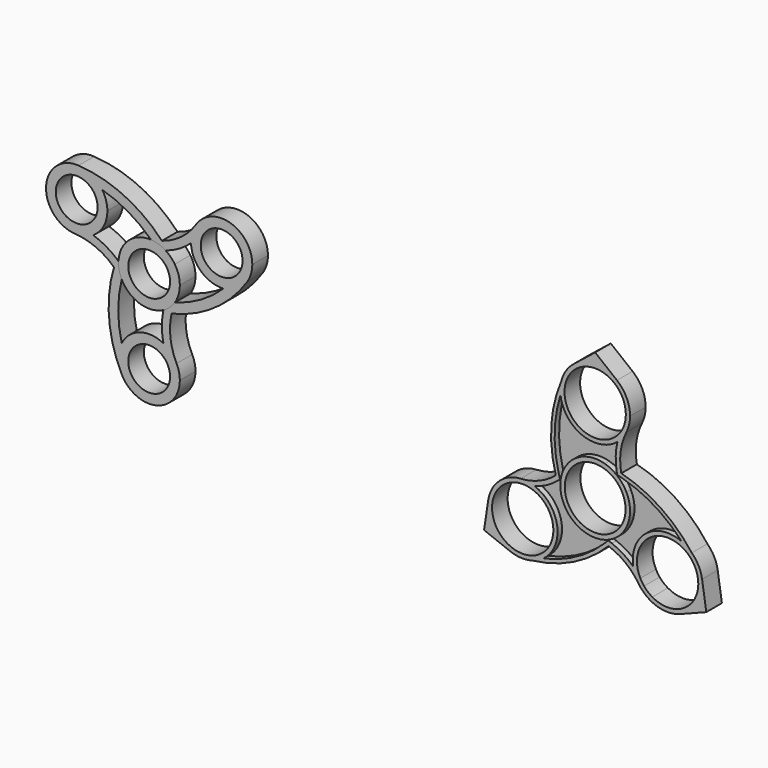
from build123d import *

# Parameters (mm, degrees)
F0_R     = 7.5
F1_DEPTH = 7
F2_DEPTH = 7
F0_R_2   = 10.9
F3_DEPTH = 5


with BuildPart() as f1:
    # F0 (on Front) → F1 (new body)
    with BuildSketch(Plane.XZ):
        with BuildLine():
            ThreePointArc((-53.6173571881, -1.7518525896), (-50.8980624665, -2.263725706), (-48.3925420942, -3.438010822))
            ThreePointArc((-48.3925420942, -3.438010822), (-48.0208333167, -3.3135242937), (-47.6510866311, -3.1833256014))
            ThreePointArc((-47.6510866311, -3.1833256014), (-48.6612372923, -1.9798547606), (-49.7132063547, -0.8127611419))
            ThreePointArc((-49.7132063547, -0.8127611419), (-51.7006557198, -1.3210314142), (-53.7260833426, -1.6465104352))
            ThreePointArc((-53.7260833426, -1.6465104352), (-53.6716717563, -1.6991314451), (-53.6173571881, -1.7518525896))
        make_face()
        with BuildLine():
            ThreePointArc((-49.7132063547, -0.8127611419), (-48.6612372923, -1.9798547606), (-47.6510866311, -3.1833256014))
            ThreePointArc((-47.6510866311, -3.1833256014), (-43.2270069865, -1.0862666914), (-39.2865137281, 1.8193571064))
            ThreePointArc((-39.2865137281, 1.8193571064), (-38.8930820127, 5.2165884842), (-37.4752941756, 8.3287978599))
            ThreePointArc((-37.4752941756, 8.3287978599), (-42.7962829401, 2.6897701484), (-49.7132063547, -0.8127611419))
        make_face()
        with BuildLine():
            ThreePointArc((-44.9512017674, -18.7514907783), (-45.0239786919, -18.7723020893), (-45.0967938264, -18.7929793129))
            ThreePointArc((-45.0967938264, -18.7929793129), (-46.8997363096, -20.8920210639), (-49.1694572375, -22.4747227981))
            ThreePointArc((-49.1694572375, -22.4747227981), (-49.2475031303, -22.8588753064), (-49.319621098, -23.2441846752))
            ThreePointArc((-49.319621098, -23.2441846752), (-47.7723094465, -22.9711039613), (-46.235592193, -22.6436188386))
            ThreePointArc((-46.235592193, -22.6436188386), (-45.6820424782, -20.6683020636), (-44.9512017674, -18.7514907783))
        make_face()
        with BuildLine():
            ThreePointArc((-27.6365950746, -8.7123288634), (-35.6733761028, -14.8021286274), (-44.9512017674, -18.7514907783))
            ThreePointArc((-44.9512017674, -18.7514907783), (-45.6820424782, -20.6683020636), (-46.235592193, -22.6436188386))
            ThreePointArc((-46.235592193, -22.6436188386), (-30.8640120209, -15.8248534989), (-19.1160317129, -3.7929793129))
            ThreePointArc((-19.1160317129, -3.7929793129), (-22.7956629442, -7.2583701681), (-27.6365950746, -8.7123288634))
        make_face()
        with BuildLine():
            ThreePointArc((-37.4752941756, 8.3287978599), (-38.8930820127, 5.2165884842), (-39.2865137281, 1.8193571064))
            ThreePointArc((-39.2865137281, 1.8193571064), (-35.6723516924, -5.8920210639), (-27.6365950746, -8.7123288634))
            ThreePointArc((-27.6365950746, -8.7123288634), (-22.7956629442, -7.2583701681), (-19.1160317129, -3.7929793129))
            ThreePointArc((-19.1160317129, -3.7929793129), (-17.7605800413, -0.8962696449), (-17.2956629442, 2.2679092735))
            ThreePointArc((-17.2956629442, 2.2679092735), (-25.1314840258, 12.8029921765), (-37.4752941756, 8.3287978599))
        make_face()
        with Locations((-28.2956629442, 2.2679092735)):
            Circle(F0_R, mode=Mode.SUBTRACT)
        with BuildLine():
            ThreePointArc((-53.7260833426, -1.6465104352), (-51.7006557198, -1.3210314142), (-49.7132063547, -0.8127611419))
            ThreePointArc((-49.7132063547, -0.8127611419), (-63.3042204474, 9.0900351135), (-79.5981193016, 13.2481474104))
            ThreePointArc((-79.5981193016, 13.2481474104), (-74.7571871713, 11.7941887151), (-71.07755594, 8.3287978599))
            ThreePointArc((-71.07755594, 8.3287978599), (-61.7852441263, 4.4136412068), (-53.7260833426, -1.6465104352))
        make_face()
        with BuildLine():
            ThreePointArc((-44.4377259568, -37.812741176), (-46.6607728253, -30.3851158769), (-46.235592193, -22.6436188386))
            ThreePointArc((-46.235592193, -22.6436188386), (-47.7723094465, -22.9711039613), (-49.319621098, -23.2441846752))
            ThreePointArc((-49.319621098, -23.2441846752), (-49.715554631, -28.1240794908), (-49.1694572375, -32.9894586549))
            ThreePointArc((-49.1694572375, -32.9894586549), (-46.4240844195, -35.028796204), (-44.4377259568, -37.812741176))
        make_face()
        with BuildLine():
            ThreePointArc((-71.07755594, 8.3287978599), (-74.7571871713, 11.7941887151), (-79.5981193016, 13.2481474104))
            ThreePointArc((-79.5981193016, 13.2481474104), (-91.2374253082, 2.9269771432), (-80.916255041, -8.7123288634))
            ThreePointArc((-80.916255041, -8.7123288634), (-77.5121087411, -8.3840644597), (-74.3733042077, -7.026170631))
            ThreePointArc((-74.3733042077, -7.026170631), (-70.6207274324, -3.0366777698), (-69.2571871713, 2.2679092735))
            ThreePointArc((-69.2571871713, 2.2679092735), (-69.7221042683, 5.4320881919), (-71.07755594, 8.3287978599))
        make_face()
        with Locations((-80.2571871713, 2.2679092735)):
            Circle(F0_R, mode=Mode.SUBTRACT)
        with BuildLine():
            ThreePointArc((-43.2764250578, -42.7320907265), (-43.5706861736, -40.2048086005), (-44.4377259568, -37.812741176))
            ThreePointArc((-44.4377259568, -37.812741176), (-46.4240844195, -35.028796204), (-49.1694572375, -32.9894586549))
            ThreePointArc((-49.1694572375, -32.9894586549), (-57.654787649, -32.263725706), (-64.1151241588, -37.812741176))
            ThreePointArc((-64.1151241588, -37.812741176), (-65.2764250578, -42.7320907265), (-64.1151241588, -47.651440277))
            ThreePointArc((-64.1151241588, -47.651440277), (-51.7491429317, -53.4378296106), (-43.2764250578, -42.7320907265))
        make_face()
        with Locations((-54.2764250578, -42.7320907265)):
            Circle(F0_R, mode=Mode.SUBTRACT)
        with BuildLine():
            ThreePointArc((-74.3733042077, -7.026170631), (-77.5121087411, -8.3840644597), (-80.916255041, -8.7123288634))
            ThreePointArc((-80.916255041, -8.7123288634), (-73.3722194079, -10.500926451), (-66.8804766256, -14.7398921989))
            ThreePointArc((-66.8804766256, -14.7398921989), (-66.3957284344, -13.2453134575), (-65.8585674442, -11.7687619029))
            ThreePointArc((-65.8585674442, -11.7687619029), (-69.8867135558, -8.9859259973), (-74.3733042077, -7.026170631))
        make_face()
        with BuildLine():
            ThreePointArc((-64.1151241588, -17.651440277), (-65.0314763972, -15.0405254095), (-65.2672758416, -12.2835385593))
            ThreePointArc((-65.2672758416, -12.2835385593), (-65.5609387263, -12.0238725794), (-65.8585674442, -11.7687619029))
            ThreePointArc((-65.8585674442, -11.7687619029), (-66.3957284344, -13.2453134575), (-66.8804766256, -14.7398921989))
            ThreePointArc((-66.8804766256, -14.7398921989), (-65.4465769753, -16.2069387016), (-64.1519900633, -17.798270966))
            ThreePointArc((-64.1519900633, -17.798270966), (-64.1336247251, -17.7248386451), (-64.1151241588, -17.651440277))
        make_face()
        with BuildLine():
            ThreePointArc((-64.1519900633, -17.798270966), (-65.4465769753, -16.2069387016), (-66.8804766256, -14.7398921989))
            ThreePointArc((-66.8804766256, -14.7398921989), (-68.6610427049, -31.4614537941), (-64.1151241588, -47.651440277))
            ThreePointArc((-64.1151241588, -47.651440277), (-65.2764250578, -42.7320907265), (-64.1151241588, -37.812741176))
            ThreePointArc((-64.1151241588, -37.812741176), (-65.3706549442, -27.8077847589), (-64.1519900633, -17.798270966))
        make_face()
        with BuildLine():
            ThreePointArc((-44.4377259568, -17.651440277), (-43.5706861736, -15.2593728525), (-43.2764250578, -12.7320907265))
            ThreePointArc((-43.2764250578, -12.7320907265), (-43.7413421548, -9.5679118081), (-45.0967938264, -6.6712021401))
            ThreePointArc((-45.0967938264, -6.6712021401), (-46.5731305353, -4.8797500882), (-48.3925420942, -3.438010822))
            ThreePointArc((-48.3925420942, -3.438010822), (-50.8980624665, -2.263725706), (-53.6173571881, -1.7518525896))
            ThreePointArc((-53.6173571881, -1.7518525896), (-54.2764250578, -1.7320907265), (-54.9354929274, -1.7518525896))
            ThreePointArc((-54.9354929274, -1.7518525896), (-60.3373136442, -3.5524594952), (-64.1151241588, -7.812741176))
            ThreePointArc((-64.1151241588, -7.812741176), (-64.9283987909, -9.9870122963), (-65.2672758416, -12.2835385593))
            ThreePointArc((-65.2672758416, -12.2835385593), (-65.0314763972, -15.0405254095), (-64.1151241588, -17.651440277))
            ThreePointArc((-64.1151241588, -17.651440277), (-63.8027044994, -18.2320907265), (-63.4560562891, -18.7929793129))
            ThreePointArc((-63.4560562891, -18.7929793129), (-59.1957746083, -22.5707898275), (-53.6173571881, -23.7123288634))
            ThreePointArc((-53.6173571881, -23.7123288634), (-51.3277458471, -23.3295097949), (-49.1694572375, -22.4747227981))
            ThreePointArc((-49.1694572375, -22.4747227981), (-46.8997363096, -20.8920210639), (-45.0967938264, -18.7929793129))
            ThreePointArc((-45.0967938264, -18.7929793129), (-44.7501456161, -18.2320907265), (-44.4377259568, -17.651440277))
        make_face()
        with Locations((-54.2764250578, -12.7320907265)):
            Circle(F0_R, mode=Mode.SUBTRACT)
    extrude(amount=F1_DEPTH)


with BuildPart() as f1b:
    # F0 (on Front) → F1, piece 2 (new body)
    with BuildSketch(Plane.XZ):
        with BuildLine():
            ThreePointArc((113.2901036685, -20.2251223841), (113.4145637461, -20.9117406905), (113.5601241099, -21.5941974218))
            ThreePointArc((113.5601241099, -21.5941974218), (114.4419800019, -21.8056031634), (115.3193491866, -22.034918482))
            ThreePointArc((115.3193491866, -22.034918482), (115.1420860534, -21.3333227671), (114.989053465, -20.6260464472))
            ThreePointArc((114.989053465, -20.6260464472), (114.141488051, -20.4174928136), (113.2901036685, -20.2251223841))
        make_face()
        with BuildLine():
            ThreePointArc((113.6417849809, -11.123598484), (113.0035342504, -15.6564929886), (113.2901036685, -20.2251223841))
            ThreePointArc((113.2901036685, -20.2251223841), (114.141488051, -20.4174928136), (114.989053465, -20.6260464472))
            ThreePointArc((114.989053465, -20.6260464472), (114.7749384437, -13.7221170116), (116.8080124932, -7.1208522234))
            ThreePointArc((116.8080124932, -7.1208522234), (117.7932836947, -4.4025953564), (118.1276708841, -1.5306857228))
            ThreePointArc((118.1276708841, -1.5306857228), (116.8949207212, 3.8821768385), (113.4398179068, 8.2274062472))
            ThreePointArc((113.4398179068, 8.2274062472), (105.6276708841, 10.9693142772), (97.8155238614, 8.2274062472))
            ThreePointArc((97.8155238614, 8.2274062472), (95.0980135598, 5.2055087987), (93.4935622624, 1.4715481048))
            ThreePointArc((93.4935622624, 1.4715481048), (89.9070791367, -13.5321823635), (91.503284962, -28.8758102311))
            ThreePointArc((91.503284962, -28.8758102311), (92.0392879282, -28.389641962), (92.558256074, -27.885329728))
            ThreePointArc((92.558256074, -27.885329728), (91.1017738419, -15.3701146731), (93.2082555904, -2.9477685578))
            ThreePointArc((93.2082555904, -2.9477685578), (100.9841034619, -13.1361707017), (113.6417849809, -11.123598484))
        make_face()
        with BuildLine():
            ThreePointArc((114.8625762594, -7.5070159271), (95.0781694948, 1.585083915), (116.6276708841, -1.5306857228))
            ThreePointArc((116.6276708841, -1.5306857228), (116.4568463207, -3.4617370849), (115.9496782727, -5.3328119005))
            ThreePointArc((115.9496782727, -5.3328119005), (115.4663699851, -6.4500352733), (114.8625762594, -7.5070159271))
        make_face(mode=Mode.SUBTRACT)
        with BuildLine():
            ThreePointArc((114.989053465, -20.6260464472), (115.1420860534, -21.3333227671), (115.3193491866, -22.034918482))
            ThreePointArc((115.3193491866, -22.034918482), (126.886084474, -27.0311753964), (136.5909109102, -35.0666151608))
            ThreePointArc((136.5909109102, -35.0666151608), (123.8795718938, -36.7064958816), (119.2936698018, -48.6746557389))
            ThreePointArc((119.2936698018, -48.6746557389), (115.6871933734, -45.85546714), (111.5873595473, -43.8193288382))
            ThreePointArc((111.5873595473, -43.8193288382), (110.9950696772, -44.4604641271), (110.3906742255, -45.0902004902))
            ThreePointArc((110.3906742255, -45.0902004902), (116.4767100133, -48.3567361602), (121.1770359922, -53.418062329))
            ThreePointArc((121.1770359922, -53.418062329), (123.0384798923, -55.6304606526), (125.3584329977, -57.3560032701))
            ThreePointArc((125.3584329977, -57.3560032701), (130.6624845644, -58.9948415932), (136.1531150248, -58.1752494876))
            ThreePointArc((136.1531150248, -58.1752494876), (142.433750545, -52.7806857228), (143.9652620475, -44.6442139281))
            ThreePointArc((143.9652620475, -44.6442139281), (142.7069772403, -40.7798322475), (140.2754980714, -37.5233563179))
            ThreePointArc((140.2754980714, -37.5233563179), (129.0751278972, -26.9155055867), (114.989053465, -20.6260464472))
        make_face()
        with BuildLine():
            ThreePointArc((142.6084329977, -46.5306857228), (137.1084329977, -56.0569651645), (126.1084329977, -56.0569651645))
            ThreePointArc((126.1084329977, -56.0569651645), (124.5215057438, -54.9435010719), (123.1546914451, -53.5687432505))
            ThreePointArc((123.1546914451, -53.5687432505), (122.4288017663, -52.5915743092), (121.8153265318, -51.5401832772))
            ThreePointArc((121.8153265318, -51.5401832772), (129.0320179617, -35.8366647035), (142.6084329977, -46.5306857228))
        make_face(mode=Mode.SUBTRACT)
        with BuildLine():
            ThreePointArc((110.3906742255, -45.0902004902), (110.9950696772, -44.4604641271), (111.5873595473, -43.8193288382))
            ThreePointArc((111.5873595473, -43.8193288382), (110.9305006125, -43.583805274), (110.2666955643, -43.3686358812))
            ThreePointArc((110.2666955643, -43.3686358812), (109.6426848757, -44.0266426153), (109.0054073918, -44.6718089585))
            ThreePointArc((109.0054073918, -44.6718089585), (109.7016386708, -44.8690924394), (110.3906742255, -45.0902004902))
        make_face()
        with BuildLine():
            ThreePointArc((93.0561929781, -29.6292238655), (92.7983477749, -28.7598113898), (92.558256074, -27.885329728))
            ThreePointArc((92.558256074, -27.885329728), (92.0392879282, -28.389641962), (91.503284962, -28.8758102311))
            ThreePointArc((91.503284962, -28.8758102311), (91.7464549242, -29.7141002277), (92.0055494366, -30.5476059461))
            ThreePointArc((92.0055494366, -30.5476059461), (92.5379482938, -30.096511204), (93.0561929781, -29.6292238655))
        make_face()
        with BuildLine():
            ThreePointArc((83.1139523186, -58.5402489554), (97.9008056186, -54.1443692183), (110.3906742255, -45.0902004902))
            ThreePointArc((110.3906742255, -45.0902004902), (109.7016386708, -44.8690924394), (109.0054073918, -44.6718089585))
            ThreePointArc((109.0054073918, -44.6718089585), (98.8951543365, -52.190767099), (87.0838461519, -56.5776734499))
            ThreePointArc((87.0838461519, -56.5776734499), (92.0193372967, -44.7493905852), (83.9475578697, -34.7938029456))
            ThreePointArc((83.9475578697, -34.7938029456), (88.1922850286, -33.0800970399), (92.0055494366, -30.5476059461))
            ThreePointArc((92.0055494366, -30.5476059461), (91.7464549242, -29.7141002277), (91.503284962, -28.8758102311))
            ThreePointArc((91.503284962, -28.8758102311), (85.6313641954, -32.5132039966), (78.897964167, -34.0531426161))
            ThreePointArc((78.897964167, -34.0531426161), (76.0512490654, -34.5590011595), (73.3969087706, -35.7053681755))
            ThreePointArc((73.3969087706, -35.7053681755), (69.3256073667, -39.4793924138), (67.2900797207, -44.6442139281))
            ThreePointArc((67.2900797207, -44.6442139281), (68.8215912233, -52.7806857228), (75.1022267434, -58.1752494876))
            ThreePointArc((75.1022267434, -58.1752494876), (79.0780218523, -59.0177337196), (83.1139523186, -58.5402489554))
        make_face()
        with BuildLine():
            ThreePointArc((90.6469087706, -46.5306857228), (74.1469087706, -56.0569651645), (74.1469087706, -37.0044062812))
            ThreePointArc((74.1469087706, -37.0044062812), (75.9046605879, -36.1868190116), (77.7786429346, -35.6905020175))
            ThreePointArc((77.7786429346, -35.6905020175), (78.9878409009, -35.5504475859), (80.2051098612, -35.5448579642))
            ThreePointArc((80.2051098612, -35.5448579642), (87.619995124, -38.9524343413), (90.6469087706, -46.5306857228))
        make_face(mode=Mode.SUBTRACT)
        with BuildLine():
            Line((145.4755362958, -54.5368615449), (143.9652620475, -44.6442139281))
            ThreePointArc((143.9652620475, -44.6442139281), (142.433750545, -52.7806857228), (136.1531150248, -58.1752494876))
            Line((136.1531150248, -58.1752494876), (145.4755362958, -54.5368615449))
        make_face()
        with BuildLine():
            ThreePointArc((97.8155238614, 8.2274062472), (105.6276708841, 10.9693142772), (113.4398179068, 8.2274062472))
            Line((113.4398179068, 8.2274062472), (105.6276708841, 14.4816659213))
            Line((105.6276708841, 14.4816659213), (97.8155238614, 8.2274062472))
        make_face()
        with BuildLine():
            Line((65.7798054725, -54.5368615449), (75.1022267434, -58.1752494876))
            ThreePointArc((75.1022267434, -58.1752494876), (68.8215912233, -52.7806857228), (67.2900797207, -44.6442139281))
            Line((67.2900797207, -44.6442139281), (65.7798054725, -54.5368615449))
        make_face()
    extrude(amount=F1_DEPTH)


with BuildPart() as f2:
    # F0 (on Front) → F2 (new body)
    with BuildSketch(Plane.XZ):
        with BuildLine():
            ThreePointArc((-53.6173571881, -1.7518525896), (-50.8980624665, -2.263725706), (-48.3925420942, -3.438010822))
            ThreePointArc((-48.3925420942, -3.438010822), (-48.0208333167, -3.3135242937), (-47.6510866311, -3.1833256014))
            ThreePointArc((-47.6510866311, -3.1833256014), (-48.6612372923, -1.9798547606), (-49.7132063547, -0.8127611419))
            ThreePointArc((-49.7132063547, -0.8127611419), (-51.7006557198, -1.3210314142), (-53.7260833426, -1.6465104352))
            ThreePointArc((-53.7260833426, -1.6465104352), (-53.6716717563, -1.6991314451), (-53.6173571881, -1.7518525896))
        make_face()
        with BuildLine():
            ThreePointArc((-49.7132063547, -0.8127611419), (-48.6612372923, -1.9798547606), (-47.6510866311, -3.1833256014))
            ThreePointArc((-47.6510866311, -3.1833256014), (-43.2270069865, -1.0862666914), (-39.2865137281, 1.8193571064))
            ThreePointArc((-39.2865137281, 1.8193571064), (-38.8930820127, 5.2165884842), (-37.4752941756, 8.3287978599))
            ThreePointArc((-37.4752941756, 8.3287978599), (-42.7962829401, 2.6897701484), (-49.7132063547, -0.8127611419))
        make_face()
        with BuildLine():
            ThreePointArc((-44.9512017674, -18.7514907783), (-45.0239786919, -18.7723020893), (-45.0967938264, -18.7929793129))
            ThreePointArc((-45.0967938264, -18.7929793129), (-46.8997363096, -20.8920210639), (-49.1694572375, -22.4747227981))
            ThreePointArc((-49.1694572375, -22.4747227981), (-49.2475031303, -22.8588753064), (-49.319621098, -23.2441846752))
            ThreePointArc((-49.319621098, -23.2441846752), (-47.7723094465, -22.9711039613), (-46.235592193, -22.6436188386))
            ThreePointArc((-46.235592193, -22.6436188386), (-45.6820424782, -20.6683020636), (-44.9512017674, -18.7514907783))
        make_face()
        with BuildLine():
            ThreePointArc((-27.6365950746, -8.7123288634), (-35.6733761028, -14.8021286274), (-44.9512017674, -18.7514907783))
            ThreePointArc((-44.9512017674, -18.7514907783), (-45.6820424782, -20.6683020636), (-46.235592193, -22.6436188386))
            ThreePointArc((-46.235592193, -22.6436188386), (-30.8640120209, -15.8248534989), (-19.1160317129, -3.7929793129))
            ThreePointArc((-19.1160317129, -3.7929793129), (-22.7956629442, -7.2583701681), (-27.6365950746, -8.7123288634))
        make_face()
        with BuildLine():
            ThreePointArc((-37.4752941756, 8.3287978599), (-38.8930820127, 5.2165884842), (-39.2865137281, 1.8193571064))
            ThreePointArc((-39.2865137281, 1.8193571064), (-35.6723516924, -5.8920210639), (-27.6365950746, -8.7123288634))
            ThreePointArc((-27.6365950746, -8.7123288634), (-22.7956629442, -7.2583701681), (-19.1160317129, -3.7929793129))
            ThreePointArc((-19.1160317129, -3.7929793129), (-17.7605800413, -0.8962696449), (-17.2956629442, 2.2679092735))
            ThreePointArc((-17.2956629442, 2.2679092735), (-25.1314840258, 12.8029921765), (-37.4752941756, 8.3287978599))
        make_face()
        with Locations((-28.2956629442, 2.2679092735)):
            Circle(F0_R, mode=Mode.SUBTRACT)
        with BuildLine():
            ThreePointArc((-53.7260833426, -1.6465104352), (-51.7006557198, -1.3210314142), (-49.7132063547, -0.8127611419))
            ThreePointArc((-49.7132063547, -0.8127611419), (-63.3042204474, 9.0900351135), (-79.5981193016, 13.2481474104))
            ThreePointArc((-79.5981193016, 13.2481474104), (-74.7571871713, 11.7941887151), (-71.07755594, 8.3287978599))
            ThreePointArc((-71.07755594, 8.3287978599), (-61.7852441263, 4.4136412068), (-53.7260833426, -1.6465104352))
        make_face()
        with BuildLine():
            ThreePointArc((-44.4377259568, -37.812741176), (-46.6607728253, -30.3851158769), (-46.235592193, -22.6436188386))
            ThreePointArc((-46.235592193, -22.6436188386), (-47.7723094465, -22.9711039613), (-49.319621098, -23.2441846752))
            ThreePointArc((-49.319621098, -23.2441846752), (-49.715554631, -28.1240794908), (-49.1694572375, -32.9894586549))
            ThreePointArc((-49.1694572375, -32.9894586549), (-46.4240844195, -35.028796204), (-44.4377259568, -37.812741176))
        make_face()
        with BuildLine():
            ThreePointArc((-71.07755594, 8.3287978599), (-74.7571871713, 11.7941887151), (-79.5981193016, 13.2481474104))
            ThreePointArc((-79.5981193016, 13.2481474104), (-91.2374253082, 2.9269771432), (-80.916255041, -8.7123288634))
            ThreePointArc((-80.916255041, -8.7123288634), (-77.5121087411, -8.3840644597), (-74.3733042077, -7.026170631))
            ThreePointArc((-74.3733042077, -7.026170631), (-70.6207274324, -3.0366777698), (-69.2571871713, 2.2679092735))
            ThreePointArc((-69.2571871713, 2.2679092735), (-69.7221042683, 5.4320881919), (-71.07755594, 8.3287978599))
        make_face()
        with Locations((-80.2571871713, 2.2679092735)):
            Circle(F0_R, mode=Mode.SUBTRACT)
        with BuildLine():
            ThreePointArc((-43.2764250578, -42.7320907265), (-43.5706861736, -40.2048086005), (-44.4377259568, -37.812741176))
            ThreePointArc((-44.4377259568, -37.812741176), (-46.4240844195, -35.028796204), (-49.1694572375, -32.9894586549))
            ThreePointArc((-49.1694572375, -32.9894586549), (-57.654787649, -32.263725706), (-64.1151241588, -37.812741176))
            ThreePointArc((-64.1151241588, -37.812741176), (-65.2764250578, -42.7320907265), (-64.1151241588, -47.651440277))
            ThreePointArc((-64.1151241588, -47.651440277), (-51.7491429317, -53.4378296106), (-43.2764250578, -42.7320907265))
        make_face()
        with Locations((-54.2764250578, -42.7320907265)):
            Circle(F0_R, mode=Mode.SUBTRACT)
        with BuildLine():
            ThreePointArc((-74.3733042077, -7.026170631), (-77.5121087411, -8.3840644597), (-80.916255041, -8.7123288634))
            ThreePointArc((-80.916255041, -8.7123288634), (-73.3722194079, -10.500926451), (-66.8804766256, -14.7398921989))
            ThreePointArc((-66.8804766256, -14.7398921989), (-66.3957284344, -13.2453134575), (-65.8585674442, -11.7687619029))
            ThreePointArc((-65.8585674442, -11.7687619029), (-69.8867135558, -8.9859259973), (-74.3733042077, -7.026170631))
        make_face()
        with BuildLine():
            ThreePointArc((-64.1151241588, -17.651440277), (-65.0314763972, -15.0405254095), (-65.2672758416, -12.2835385593))
            ThreePointArc((-65.2672758416, -12.2835385593), (-65.5609387263, -12.0238725794), (-65.8585674442, -11.7687619029))
            ThreePointArc((-65.8585674442, -11.7687619029), (-66.3957284344, -13.2453134575), (-66.8804766256, -14.7398921989))
            ThreePointArc((-66.8804766256, -14.7398921989), (-65.4465769753, -16.2069387016), (-64.1519900633, -17.798270966))
            ThreePointArc((-64.1519900633, -17.798270966), (-64.1336247251, -17.7248386451), (-64.1151241588, -17.651440277))
        make_face()
        with BuildLine():
            ThreePointArc((-64.1519900633, -17.798270966), (-65.4465769753, -16.2069387016), (-66.8804766256, -14.7398921989))
            ThreePointArc((-66.8804766256, -14.7398921989), (-68.6610427049, -31.4614537941), (-64.1151241588, -47.651440277))
            ThreePointArc((-64.1151241588, -47.651440277), (-65.2764250578, -42.7320907265), (-64.1151241588, -37.812741176))
            ThreePointArc((-64.1151241588, -37.812741176), (-65.3706549442, -27.8077847589), (-64.1519900633, -17.798270966))
        make_face()
    extrude(amount=F2_DEPTH)


with BuildPart() as f2b:
    # F0 (on Front) → F2, piece 2 (new body)
    with BuildSketch(Plane.XZ):
        with BuildLine():
            ThreePointArc((113.2901036685, -20.2251223841), (113.4145637461, -20.9117406905), (113.5601241099, -21.5941974218))
            ThreePointArc((113.5601241099, -21.5941974218), (114.4419800019, -21.8056031634), (115.3193491866, -22.034918482))
            ThreePointArc((115.3193491866, -22.034918482), (115.1420860534, -21.3333227671), (114.989053465, -20.6260464472))
            ThreePointArc((114.989053465, -20.6260464472), (114.141488051, -20.4174928136), (113.2901036685, -20.2251223841))
        make_face()
        with BuildLine():
            ThreePointArc((113.6417849809, -11.123598484), (113.0035342504, -15.6564929886), (113.2901036685, -20.2251223841))
            ThreePointArc((113.2901036685, -20.2251223841), (114.141488051, -20.4174928136), (114.989053465, -20.6260464472))
            ThreePointArc((114.989053465, -20.6260464472), (114.7749384437, -13.7221170116), (116.8080124932, -7.1208522234))
            ThreePointArc((116.8080124932, -7.1208522234), (117.7932836947, -4.4025953564), (118.1276708841, -1.5306857228))
            ThreePointArc((118.1276708841, -1.5306857228), (116.8949207212, 3.8821768385), (113.4398179068, 8.2274062472))
            ThreePointArc((113.4398179068, 8.2274062472), (105.6276708841, 10.9693142772), (97.8155238614, 8.2274062472))
            ThreePointArc((97.8155238614, 8.2274062472), (95.0980135598, 5.2055087987), (93.4935622624, 1.4715481048))
            ThreePointArc((93.4935622624, 1.4715481048), (89.9070791367, -13.5321823635), (91.503284962, -28.8758102311))
            ThreePointArc((91.503284962, -28.8758102311), (92.0392879282, -28.389641962), (92.558256074, -27.885329728))
            ThreePointArc((92.558256074, -27.885329728), (91.1017738419, -15.3701146731), (93.2082555904, -2.9477685578))
            ThreePointArc((93.2082555904, -2.9477685578), (100.9841034619, -13.1361707017), (113.6417849809, -11.123598484))
        make_face()
        with BuildLine():
            ThreePointArc((114.8625762594, -7.5070159271), (95.0781694948, 1.585083915), (116.6276708841, -1.5306857228))
            ThreePointArc((116.6276708841, -1.5306857228), (116.4568463207, -3.4617370849), (115.9496782727, -5.3328119005))
            ThreePointArc((115.9496782727, -5.3328119005), (115.4663699851, -6.4500352733), (114.8625762594, -7.5070159271))
        make_face(mode=Mode.SUBTRACT)
        with BuildLine():
            ThreePointArc((114.989053465, -20.6260464472), (115.1420860534, -21.3333227671), (115.3193491866, -22.034918482))
            ThreePointArc((115.3193491866, -22.034918482), (126.886084474, -27.0311753964), (136.5909109102, -35.0666151608))
            ThreePointArc((136.5909109102, -35.0666151608), (123.8795718938, -36.7064958816), (119.2936698018, -48.6746557389))
            ThreePointArc((119.2936698018, -48.6746557389), (115.6871933734, -45.85546714), (111.5873595473, -43.8193288382))
            ThreePointArc((111.5873595473, -43.8193288382), (110.9950696772, -44.4604641271), (110.3906742255, -45.0902004902))
            ThreePointArc((110.3906742255, -45.0902004902), (116.4767100133, -48.3567361602), (121.1770359922, -53.418062329))
            ThreePointArc((121.1770359922, -53.418062329), (123.0384798923, -55.6304606526), (125.3584329977, -57.3560032701))
            ThreePointArc((125.3584329977, -57.3560032701), (130.6624845644, -58.9948415932), (136.1531150248, -58.1752494876))
            ThreePointArc((136.1531150248, -58.1752494876), (142.433750545, -52.7806857228), (143.9652620475, -44.6442139281))
            ThreePointArc((143.9652620475, -44.6442139281), (142.7069772403, -40.7798322475), (140.2754980714, -37.5233563179))
            ThreePointArc((140.2754980714, -37.5233563179), (129.0751278972, -26.9155055867), (114.989053465, -20.6260464472))
        make_face()
        with BuildLine():
            ThreePointArc((142.6084329977, -46.5306857228), (137.1084329977, -56.0569651645), (126.1084329977, -56.0569651645))
            ThreePointArc((126.1084329977, -56.0569651645), (124.5215057438, -54.9435010719), (123.1546914451, -53.5687432505))
            ThreePointArc((123.1546914451, -53.5687432505), (122.4288017663, -52.5915743092), (121.8153265318, -51.5401832772))
            ThreePointArc((121.8153265318, -51.5401832772), (129.0320179617, -35.8366647035), (142.6084329977, -46.5306857228))
        make_face(mode=Mode.SUBTRACT)
        with BuildLine():
            ThreePointArc((110.3906742255, -45.0902004902), (110.9950696772, -44.4604641271), (111.5873595473, -43.8193288382))
            ThreePointArc((111.5873595473, -43.8193288382), (110.9305006125, -43.583805274), (110.2666955643, -43.3686358812))
            ThreePointArc((110.2666955643, -43.3686358812), (109.6426848757, -44.0266426153), (109.0054073918, -44.6718089585))
            ThreePointArc((109.0054073918, -44.6718089585), (109.7016386708, -44.8690924394), (110.3906742255, -45.0902004902))
        make_face()
        with BuildLine():
            ThreePointArc((93.0561929781, -29.6292238655), (92.7983477749, -28.7598113898), (92.558256074, -27.885329728))
            ThreePointArc((92.558256074, -27.885329728), (92.0392879282, -28.389641962), (91.503284962, -28.8758102311))
            ThreePointArc((91.503284962, -28.8758102311), (91.7464549242, -29.7141002277), (92.0055494366, -30.5476059461))
            ThreePointArc((92.0055494366, -30.5476059461), (92.5379482938, -30.096511204), (93.0561929781, -29.6292238655))
        make_face()
        with BuildLine():
            ThreePointArc((83.1139523186, -58.5402489554), (97.9008056186, -54.1443692183), (110.3906742255, -45.0902004902))
            ThreePointArc((110.3906742255, -45.0902004902), (109.7016386708, -44.8690924394), (109.0054073918, -44.6718089585))
            ThreePointArc((109.0054073918, -44.6718089585), (98.8951543365, -52.190767099), (87.0838461519, -56.5776734499))
            ThreePointArc((87.0838461519, -56.5776734499), (92.0193372967, -44.7493905852), (83.9475578697, -34.7938029456))
            ThreePointArc((83.9475578697, -34.7938029456), (88.1922850286, -33.0800970399), (92.0055494366, -30.5476059461))
            ThreePointArc((92.0055494366, -30.5476059461), (91.7464549242, -29.7141002277), (91.503284962, -28.8758102311))
            ThreePointArc((91.503284962, -28.8758102311), (85.6313641954, -32.5132039966), (78.897964167, -34.0531426161))
            ThreePointArc((78.897964167, -34.0531426161), (76.0512490654, -34.5590011595), (73.3969087706, -35.7053681755))
            ThreePointArc((73.3969087706, -35.7053681755), (69.3256073667, -39.4793924138), (67.2900797207, -44.6442139281))
            ThreePointArc((67.2900797207, -44.6442139281), (68.8215912233, -52.7806857228), (75.1022267434, -58.1752494876))
            ThreePointArc((75.1022267434, -58.1752494876), (79.0780218523, -59.0177337196), (83.1139523186, -58.5402489554))
        make_face()
        with BuildLine():
            ThreePointArc((90.6469087706, -46.5306857228), (74.1469087706, -56.0569651645), (74.1469087706, -37.0044062812))
            ThreePointArc((74.1469087706, -37.0044062812), (75.9046605879, -36.1868190116), (77.7786429346, -35.6905020175))
            ThreePointArc((77.7786429346, -35.6905020175), (78.9878409009, -35.5504475859), (80.2051098612, -35.5448579642))
            ThreePointArc((80.2051098612, -35.5448579642), (87.619995124, -38.9524343413), (90.6469087706, -46.5306857228))
        make_face(mode=Mode.SUBTRACT)
        with BuildLine():
            Line((145.4755362958, -54.5368615449), (143.9652620475, -44.6442139281))
            ThreePointArc((143.9652620475, -44.6442139281), (142.433750545, -52.7806857228), (136.1531150248, -58.1752494876))
            Line((136.1531150248, -58.1752494876), (145.4755362958, -54.5368615449))
        make_face()
        with BuildLine():
            ThreePointArc((97.8155238614, 8.2274062472), (105.6276708841, 10.9693142772), (113.4398179068, 8.2274062472))
            Line((113.4398179068, 8.2274062472), (105.6276708841, 14.4816659213))
            Line((105.6276708841, 14.4816659213), (97.8155238614, 8.2274062472))
        make_face()
        with BuildLine():
            Line((65.7798054725, -54.5368615449), (75.1022267434, -58.1752494876))
            ThreePointArc((75.1022267434, -58.1752494876), (68.8215912233, -52.7806857228), (67.2900797207, -44.6442139281))
            Line((67.2900797207, -44.6442139281), (65.7798054725, -54.5368615449))
        make_face()
    extrude(amount=F2_DEPTH)


with BuildPart() as f2c:
    # F0 (on Front) → F2, piece 3 (new body)
    with BuildSketch(Plane.XZ):
        with BuildLine():
            ThreePointArc((116.8080107716, -25.9405157791), (115.4313565918, -23.7758326265), (113.6417849809, -21.9377729616))
            ThreePointArc((113.6417849809, -21.9377729616), (113.356531988, -21.7064958816), (113.0646082654, -21.4836979958))
            ThreePointArc((113.0646082654, -21.4836979958), (111.16726705, -20.3252016048), (109.0947144322, -19.5211224903))
            ThreePointArc((109.0947144322, -19.5211224903), (101.3050826153, -19.8018652085), (95.1962717576, -24.6433123292))
            ThreePointArc((95.1962717576, -24.6433123292), (94.0099282463, -26.9178713975), (93.3129076883, -29.3867157068))
            ThreePointArc((93.3129076883, -29.3867157068), (93.2552423581, -29.7493905852), (93.2082555904, -30.1136028878))
            ThreePointArc((93.2082555904, -30.1136028878), (93.1536388933, -32.3359967755), (93.4935622624, -34.5329195505))
            ThreePointArc((93.4935622624, -34.5329195505), (97.6315084967, -41.1385672309), (104.8787301231, -44.0082290602))
            ThreePointArc((104.8787301231, -44.0082290602), (107.4417278144, -43.8983531445), (109.9283199832, -43.2675685001))
            ThreePointArc((109.9283199832, -43.2675685001), (110.2712383063, -43.1361707017), (110.6101487966, -42.9947562849))
            ThreePointArc((110.6101487966, -42.9947562849), (112.5621067091, -41.9308587882), (114.2947359578, -40.5380151277))
            ThreePointArc((114.2947359578, -40.5380151277), (117.9464215404, -33.6516247291), (116.8080107716, -25.9405157791))
        make_face()
        with Locations((105.6276708841, -31.5306857228)):
            Circle(F0_R_2, mode=Mode.SUBTRACT)
    extrude(amount=F2_DEPTH)


with BuildPart() as f3:
    # F0 (on Front) → F3 (new body)
    with BuildSketch(Plane.XZ):
        with BuildLine():
            ThreePointArc((113.5601241099, -21.5941974218), (113.6002846637, -21.7661444089), (113.6417849809, -21.9377729616))
            ThreePointArc((113.6417849809, -21.9377729616), (115.4313565918, -23.7758326265), (116.8080107716, -25.9405157791))
            ThreePointArc((116.8080107716, -25.9405157791), (115.9664612903, -24.0247731085), (115.3193491866, -22.034918482))
            ThreePointArc((115.3193491866, -22.034918482), (114.4419800019, -21.8056031634), (113.5601241099, -21.5941974218))
        make_face()
        with BuildLine():
            ThreePointArc((115.3193491866, -22.034918482), (115.9664612903, -24.0247731085), (116.8080107716, -25.9405157791))
            ThreePointArc((116.8080107716, -25.9405157791), (117.9464215404, -33.6516247291), (114.2947359578, -40.5380151277))
            ThreePointArc((114.2947359578, -40.5380151277), (112.9791499731, -42.2101097125), (111.5873595473, -43.8193288382))
            ThreePointArc((111.5873595473, -43.8193288382), (115.6871933734, -45.85546714), (119.2936698018, -48.6746557389))
            ThreePointArc((119.2936698018, -48.6746557389), (123.8795718938, -36.7064958816), (136.5909109102, -35.0666151608))
            ThreePointArc((136.5909109102, -35.0666151608), (126.886084474, -27.0311753964), (115.3193491866, -22.034918482))
        make_face()
        with BuildLine():
            ThreePointArc((111.5873595473, -43.8193288382), (112.9791499731, -42.2101097125), (114.2947359578, -40.5380151277))
            ThreePointArc((114.2947359578, -40.5380151277), (112.5621067091, -41.9308587882), (110.6101487966, -42.9947562849))
            ThreePointArc((110.6101487966, -42.9947562849), (110.4389548786, -43.1821854301), (110.2666955643, -43.3686358812))
            ThreePointArc((110.2666955643, -43.3686358812), (110.9305006125, -43.583805274), (111.5873595473, -43.8193288382))
        make_face()
    extrude(amount=F3_DEPTH)


with BuildPart() as f3b:
    # F0 (on Front) → F3, piece 2 (new body)
    with BuildSketch(Plane.XZ):
        with BuildLine():
            ThreePointArc((109.0947144322, -19.5211224903), (111.16726705, -20.3252016048), (113.0646082654, -21.4836979958))
            ThreePointArc((113.0646082654, -21.4836979958), (113.3125236256, -21.5382417051), (113.5601241099, -21.5941974218))
            ThreePointArc((113.5601241099, -21.5941974218), (113.4145637461, -20.9117406905), (113.2901036685, -20.2251223841))
            ThreePointArc((113.2901036685, -20.2251223841), (111.2005838125, -19.8244060816), (109.0947144322, -19.5211224903))
        make_face()
        with BuildLine():
            ThreePointArc((95.1962717576, -24.6433123292), (101.3050826153, -19.8018652085), (109.0947144322, -19.5211224903))
            ThreePointArc((109.0947144322, -19.5211224903), (111.2005838125, -19.8244060816), (113.2901036685, -20.2251223841))
            ThreePointArc((113.2901036685, -20.2251223841), (113.0035342504, -15.6564929886), (113.6417849809, -11.123598484))
            ThreePointArc((113.6417849809, -11.123598484), (100.9841034619, -13.1361707017), (93.2082555904, -2.9477685578))
            ThreePointArc((93.2082555904, -2.9477685578), (91.1017738419, -15.3701146731), (92.558256074, -27.885329728))
            ThreePointArc((92.558256074, -27.885329728), (93.9579646785, -26.3299868938), (95.1962717576, -24.6433123292))
        make_face()
        with BuildLine():
            ThreePointArc((93.3129076883, -29.3867157068), (94.0099282463, -26.9178713975), (95.1962717576, -24.6433123292))
            ThreePointArc((95.1962717576, -24.6433123292), (93.9579646785, -26.3299868938), (92.558256074, -27.885329728))
            ThreePointArc((92.558256074, -27.885329728), (92.7983477749, -28.7598113898), (93.0561929781, -29.6292238655))
            ThreePointArc((93.0561929781, -29.6292238655), (93.1850231602, -29.5084703121), (93.3129076883, -29.3867157068))
        make_face()
    extrude(amount=F3_DEPTH)


with BuildPart() as f3c:
    # F0 (on Front) → F3, piece 3 (new body)
    with BuildSketch(Plane.XZ):
        with BuildLine():
            ThreePointArc((110.2666955643, -43.3686358812), (110.0977048285, -43.3174424475), (109.9283199832, -43.2675685001))
            ThreePointArc((109.9283199832, -43.2675685001), (107.4417278144, -43.8983531445), (104.8787301231, -44.0082290602))
            ThreePointArc((104.8787301231, -44.0082290602), (106.9585866836, -44.2372971661), (109.0054073918, -44.6718089585))
            ThreePointArc((109.0054073918, -44.6718089585), (109.6426848757, -44.0266426153), (110.2666955643, -43.3686358812))
        make_face()
        with BuildLine():
            ThreePointArc((93.4935622624, -34.5329195505), (93.1536388933, -32.3359967755), (93.2082555904, -30.1136028878))
            ThreePointArc((93.2082555904, -30.1136028878), (93.1315341482, -29.8716300332), (93.0561929781, -29.6292238655))
            ThreePointArc((93.0561929781, -29.6292238655), (92.5379482938, -30.096511204), (92.0055494366, -30.5476059461))
            ThreePointArc((92.0055494366, -30.5476059461), (92.7032788668, -32.5575413744), (93.4935622624, -34.5329195505))
        make_face()
        with BuildLine():
            ThreePointArc((109.0054073918, -44.6718089585), (106.9585866836, -44.2372971661), (104.8787301231, -44.0082290602))
            ThreePointArc((104.8787301231, -44.0082290602), (97.6315084967, -41.1385672309), (93.4935622624, -34.5329195505))
            ThreePointArc((93.4935622624, -34.5329195505), (92.7032788668, -32.5575413744), (92.0055494366, -30.5476059461))
            ThreePointArc((92.0055494366, -30.5476059461), (88.1922850286, -33.0800970399), (83.9475578697, -34.7938029456))
            ThreePointArc((83.9475578697, -34.7938029456), (92.0193372967, -44.7493905852), (87.0838461519, -56.5776734499))
            ThreePointArc((87.0838461519, -56.5776734499), (98.8951543365, -52.190767099), (109.0054073918, -44.6718089585))
        make_face()
    extrude(amount=F3_DEPTH)


solid = Compound([f1.part, f1b.part, f2.part, f2b.part, f2c.part, f3.part, f3b.part, f3c.part])
